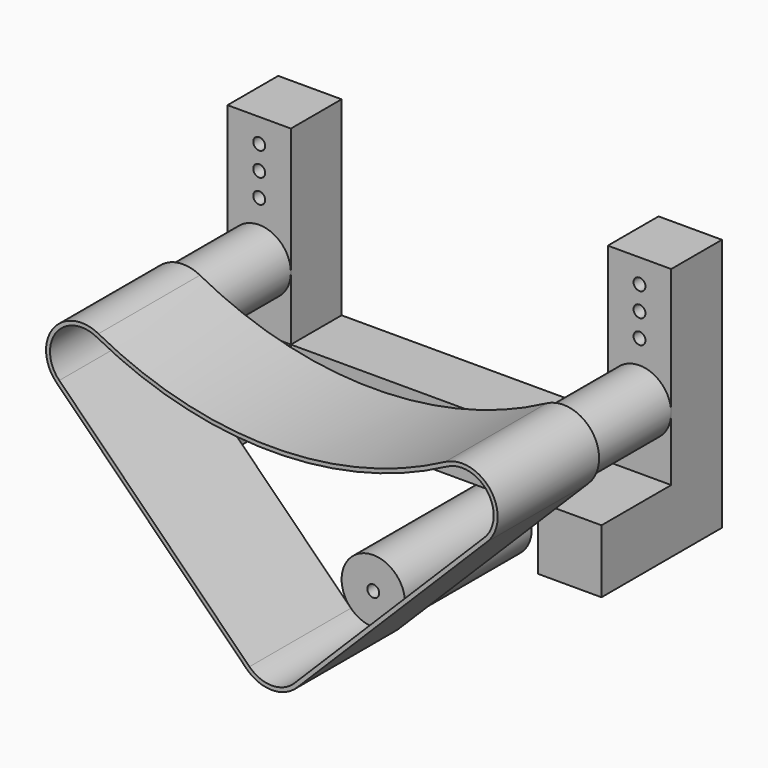
from build123d import *

# Parameters (mm, degrees)
F0_R     = 50.8
F0_R_2   = 9.525
F1_DEPTH = 254
F2_R     = 9.525
F3_DEPTH = 101.6
F5_DEPTH = 203.2
F6_W     = 101.6
F6_H     = 101.6
F7_DEPTH = 139.7


# Not quite as in the source:
# - a feature names something its author has since deleted; it is built from what else it names


with BuildPart() as f1:
    # F0 (on Front) → F1 (new body)
    with BuildSketch(Plane.XZ):
        with Locations((-304.8, 0)):
            Circle(F0_R)
        with Locations((-304.8, 0)):
            Circle(F0_R_2, mode=Mode.SUBTRACT)
    extrude(amount=F1_DEPTH)


with BuildPart() as f1b:
    # F0 (on Front) → F1, piece 2 (new body)
    with BuildSketch(Plane.XZ):
        with Locations((304.8, 0)):
            Circle(F0_R)
        with Locations((304.8, 0)):
            Circle(F0_R_2, mode=Mode.SUBTRACT)
    extrude(amount=F1_DEPTH)


with BuildPart() as f1c:
    # F0 (on Front) → F1, piece 3 (new body)
    with BuildSketch(Plane.XZ):
        with Locations((0, -304.8)):
            Circle(F0_R)
        with Locations((0, -304.8)):
            Circle(F0_R_2, mode=Mode.SUBTRACT)
    extrude(amount=F1_DEPTH)


with BuildPart() as f3:
    # F2 (on Front) → F3 (new body)
    with BuildSketch(Plane.XZ):
        Polygon((-254, 203.2), (-287.8666666667, 203.2), (-321.7333333333, 203.2), (-355.6, 203.2), (-355.6, -203.2), (355.6, -203.2), (355.6, 203.2), (254, 203.2), (254, -101.6), (-254, -101.6), align=None)
        with Locations((0, -139.7)):
            Circle(F2_R, mode=Mode.SUBTRACT)
        with Locations((-304.8, 88.9)):
            Circle(F2_R, mode=Mode.SUBTRACT)
        with Locations((-304.8, 127)):
            Circle(F2_R, mode=Mode.SUBTRACT)
        with Locations((-304.8, 165.1)):
            Circle(F2_R, mode=Mode.SUBTRACT)
        with Locations((304.8, 88.9)):
            Circle(F2_R, mode=Mode.SUBTRACT)
        with Locations((304.8, 127)):
            Circle(F2_R, mode=Mode.SUBTRACT)
        with Locations((304.8, 165.1)):
            Circle(F2_R, mode=Mode.SUBTRACT)
    extrude(amount=F3_DEPTH)

    # F6 (on face) → F7 (join)
    with BuildSketch(Plane.XZ.offset(101.6)):
        with Locations((-304.8, -152.4)):
            Rectangle(F6_W, F6_H)
        with Locations((304.8, -152.4)):
            Rectangle(F6_W, F6_H)
    extrude(amount=F7_DEPTH)


with BuildPart() as f5:
    # F4 (on face) → F5 (new body)
    with BuildSketch(Plane.XZ.offset(254)):
        with BuildLine():
            ThreePointArc((277.8891748053, 50.4175563404), (0, -19.1036567568), (-277.8891748053, 50.4175563404))
            ThreePointArc((-277.8891748053, 50.4175563404), (-350.7132693138, 34.030783137), (-345.2111525448, -40.4111525448))
            Line((-345.2111525448, -40.4111525448), (-40.4111525448, -345.2111525448))
            ThreePointArc((-40.4111525448, -345.2111525448), (0, -361.95), (40.4111525448, -345.2111525448))
            Line((40.4111525448, -345.2111525448), (345.2111525448, -40.4111525448))
            ThreePointArc((345.2111525448, -40.4111525448), (350.7132693138, 34.030783137), (277.8891748053, 50.4175563404))
        make_face()
        with BuildLine():
            ThreePointArc((-340.7210244843, -35.9210244843), (-345.6117949456, 30.2495850107), (-280.8792664936, 44.8156056359))
            ThreePointArc((-280.8792664936, 44.8156056359), (0, -25.4536567568), (280.8792664936, 44.8156056359))
            ThreePointArc((280.8792664936, 44.8156056359), (345.6117949456, 30.2495850107), (340.7210244843, -35.9210244843))
            Line((340.7210244843, -35.9210244843), (35.9210244843, -340.7210244843))
            ThreePointArc((35.9210244843, -340.7210244843), (0, -355.6), (-35.9210244843, -340.7210244843))
            Line((-35.9210244843, -340.7210244843), (-340.7210244843, -35.9210244843))
        make_face(mode=Mode.SUBTRACT)
    extrude(amount=F5_DEPTH)


solid = Compound([f1.part, f1b.part, f1c.part, f3.part, f5.part])
